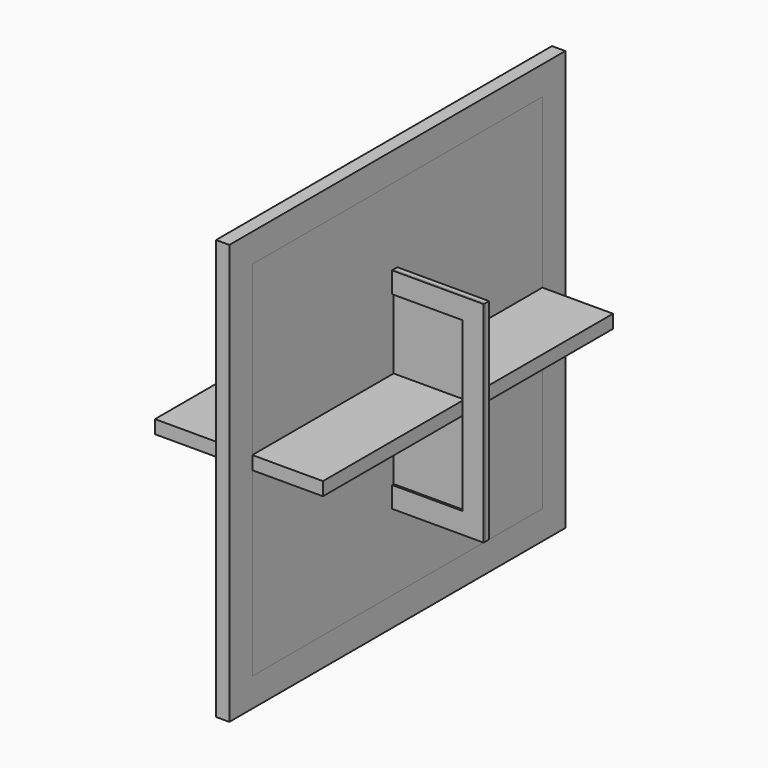
from build123d import *

# Parameters (mm, degrees)
F0_W      = 50
F0_H      = 50
F0_W_2    = 40
F0_H_2    = 40
F1_DEPTH  = 1.5875
F2_W      = 100
F2_H      = 100
F2_R      = 3.175
F2_W_2    = 40
F2_H_2    = 40
F3_DEPTH  = 3.175
F4_W      = 40
F4_H      = 80
F5_DEPTH  = 3.175
F6_W      = 50
F6_H      = 50
F7_DEPTH  = 1.1
F8_W      = 40
F8_H      = 86.35
F9_DEPTH  = 3.175
F10_W     = 86.35
F10_H     = 86.35
F11_DEPTH = 3.175


# Not quite as in the source:
# - a length typed as a fraction of an inch, garbled in the dataset ("3 / 203.2 mm" for 3/8 in), is restored


with BuildPart() as f1:
    # F0 (on Front) → F1 (new body)
    with BuildSketch(Plane.XZ):
        Rectangle(F0_W, F0_H)
        Rectangle(F0_W_2, F0_H_2, mode=Mode.SUBTRACT)
    extrude(amount=F1_DEPTH)


with BuildPart() as f3:
    # F2 (on Right) → F3 (new body)
    with BuildSketch(Plane.YZ):
        Rectangle(F2_W, F2_H)
        with Locations((-40, -40)):
            Circle(F2_R, mode=Mode.SUBTRACT)
        with Locations((40, -40)):
            Circle(F2_R, mode=Mode.SUBTRACT)
        with Locations((-40, 40)):
            Circle(F2_R, mode=Mode.SUBTRACT)
        Rectangle(F2_W_2, F2_H_2, mode=Mode.SUBTRACT)
        with Locations((40, 40)):
            Circle(F2_R, mode=Mode.SUBTRACT)
    extrude(amount=F3_DEPTH)


with BuildPart() as f5:
    # F4 (on Top) → F5 (new body)
    with BuildSketch(Plane.XY):
        Rectangle(F4_W, F4_H)
    extrude(amount=F5_DEPTH)


with BuildPart() as f7:
    # F6 (on Front) → F7 (new body)
    with BuildSketch(Plane.XZ):
        Rectangle(F6_W, F6_H)
    extrude(amount=F7_DEPTH)


with BuildPart() as f9:
    # F8 (on Top) → F9 (new body)
    with BuildSketch(Plane.XY):
        Rectangle(F8_W, F8_H)
    extrude(amount=F9_DEPTH)


with BuildPart() as f11:
    # F10 (on Right) → F11 (new body)
    with BuildSketch(Plane.YZ):
        Rectangle(F10_W, F10_H)
    extrude(amount=F11_DEPTH)


solid = Compound([f1.part, f3.part, f5.part, f7.part, f9.part, f11.part])
